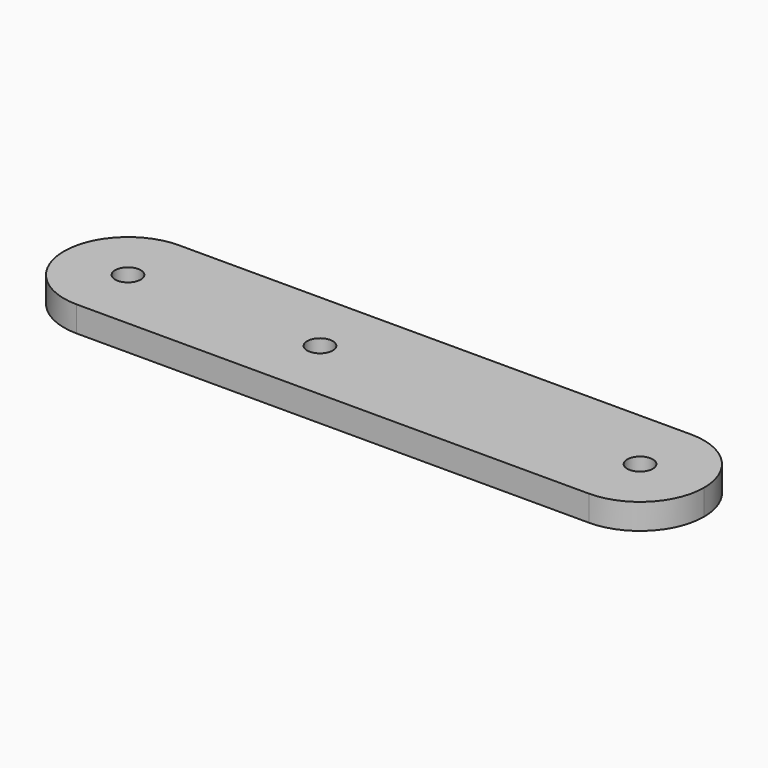
from build123d import *

# Parameters (mm, degrees)
F0_W     = 50
F0_H     = 10
F0_R     = 1
F1_DEPTH = 2
F2_R     = 4.99999


# Not quite as in the source:
# - a fillet or chamfer is up to 0.001 mm smaller than in the source, because OpenCascade refuses the exact size


with BuildPart() as f1:
    # F0 (on Top) → F1 (new body)
    with BuildSketch(Plane.XY):
        with Locations((25, -5)):
            Rectangle(F0_W, F0_H)
        with Locations((5, -5)):
            Circle(F0_R, mode=Mode.SUBTRACT)
        with Locations((20, -5)):
            Circle(F0_R, mode=Mode.SUBTRACT)
        with Locations((45, -5)):
            Circle(F0_R, mode=Mode.SUBTRACT)
    extrude(amount=F1_DEPTH)

    # F2 (radius 5 in the source; OpenCascade refuses exactly that, so slightly less here)
    f2_edges = [f1.edges().sort_by_distance(p)[0] for p in [
        (0, 0, 1),
        (0, -10, 1),
        (50, 0, 1),
        (50, -10, 1),
    ]]
    fillet(f2_edges, radius=F2_R)


solid = f1.part
